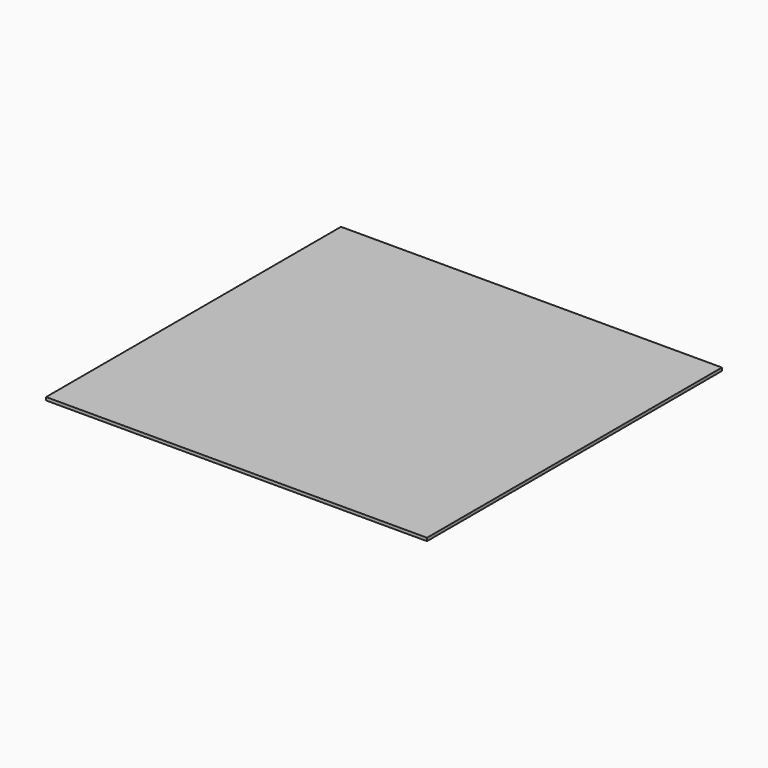
from build123d import *

# Parameters (mm, degrees)
F0_W     = 1574.8
F0_H     = 1524
F1_DEPTH = 12.7


# Not quite as in the source:
# - a length typed as a fraction of an inch, garbled in the dataset ("3 / 203.2 mm" for 3/8 in), is restored


with BuildPart() as f1:
    # F0 (on Top) → F1 (new body)
    with BuildSketch(Plane.XY):
        with Locations((-7.5279446319, -24.1771063544)):
            Rectangle(F0_W, F0_H)
    extrude(amount=F1_DEPTH)


solid = f1.part
